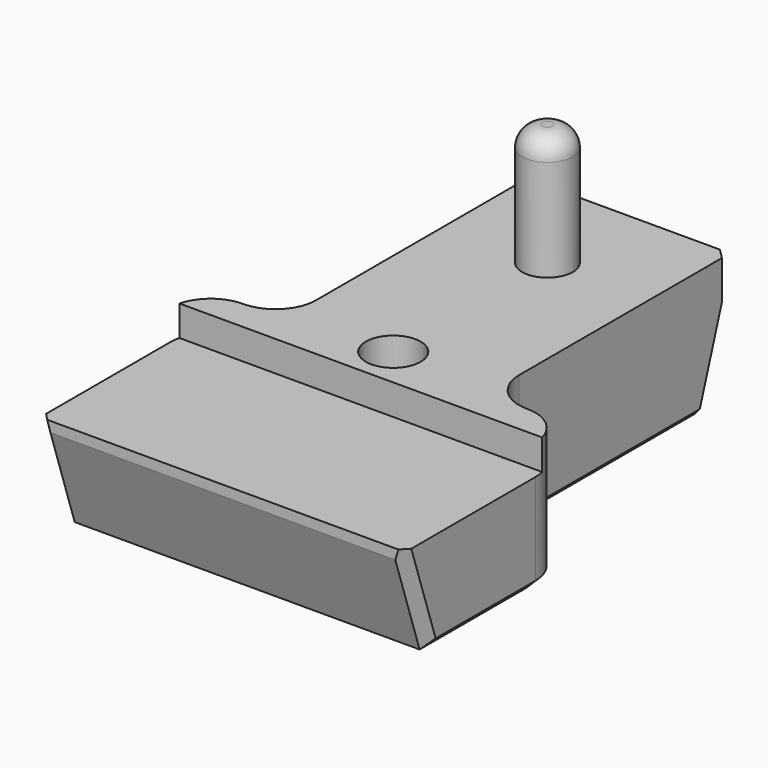
from build123d import *

# Parameters (mm, degrees)
F0_W     = 20
F0_H     = 30
F0_R     = 2.5
F1_DEPTH = 13
F2_W     = 36
F2_H     = 17
F3_DEPTH = 3
F4_D     = 5.4
F5_DEPTH = 25
F6_R     = 2
F7_R     = 3.99999
F8_SIZE2 = 9
F8_SIZE  = 3
F9_SIZE  = 1


# Not quite as in the source:
# - a fillet or chamfer is up to 0.001 mm smaller than in the source, because OpenCascade refuses the exact size


with BuildPart() as f1:
    # F0 (on Top) → F1 (new body)
    with BuildSketch(Plane.XY):
        Polygon((-18, 20), (-18, 0), (18, 0), (18, 20), (10, 20), (-10, 20), align=None)
        with Locations((0, 35)):
            Rectangle(F0_W, F0_H)
        with Locations((0, 40)):
            Circle(F0_R, mode=Mode.SUBTRACT)
        with Locations((0, 40)):
            Circle(F0_R)
    extrude(amount=F1_DEPTH)

    # F2 (on face) → F3 (cut)
    with BuildSketch(Plane.XY.offset(13)):
        with Locations((0, 8.5)):
            Rectangle(F2_W, F2_H)
    extrude(amount=-F3_DEPTH, mode=Mode.SUBTRACT)

    # F4 (through all)
    with Locations(Plane(origin=(0, 0, 0), x_dir=(1, 0, 0), z_dir=(0, 0, -1))):
        with Locations((0, -21)):
            Hole(F4_D / 2)

    # F0 (on Top) → F5 (join)
    with BuildSketch(Plane.XY):
        with Locations((0, 40)):
            Circle(F0_R)
    extrude(amount=F5_DEPTH)

    # F6
    f6_edges = [f1.edges().sort_by_distance(p)[0] for p in [
        (-2.5, 40, 25),
    ]]
    fillet(f6_edges, radius=F6_R)

    # F7 (radius 4 in the source; OpenCascade refuses exactly that, so slightly less here)
    f7_edges = [f1.edges().sort_by_distance(p)[0] for p in [
        (-18, 20, 6.5),
        (18, 20, 6.5),
        (-10, 20, 6.5),
        (10, 20, 6.5),
    ]]
    fillet(f7_edges, radius=F7_R)

    # F8
    f8_edges = [f1.edges().sort_by_distance(p)[0] for p in [
        (0, 50, 0),
        (0, 0, 0),
    ]]
    f8_side = f1.faces().sort_by_distance((-17.383883, 8.000005, 0))[0]
    chamfer(f8_edges, length=F8_SIZE, length2=F8_SIZE2, reference=f8_side)

    # F9
    f9_edges = [f1.edges().sort_by_distance(p)[0] for p in [
        (16.82843, 18.82843, 0),
        (11.17157, 21.17157, 0),
        (-11.17157, 21.17157, 0),
        (-16.82843, 18.82843, 0),
        (18, 1.5, 4.5),
        (-18, 1.5, 4.5),
        (-10, 50, 11),
        (-10, 48.5, 4.5),
        (10, 50, 11),
        (10, 48.5, 4.5),
    ]]
    chamfer(f9_edges, length=F9_SIZE)


solid = f1.part
